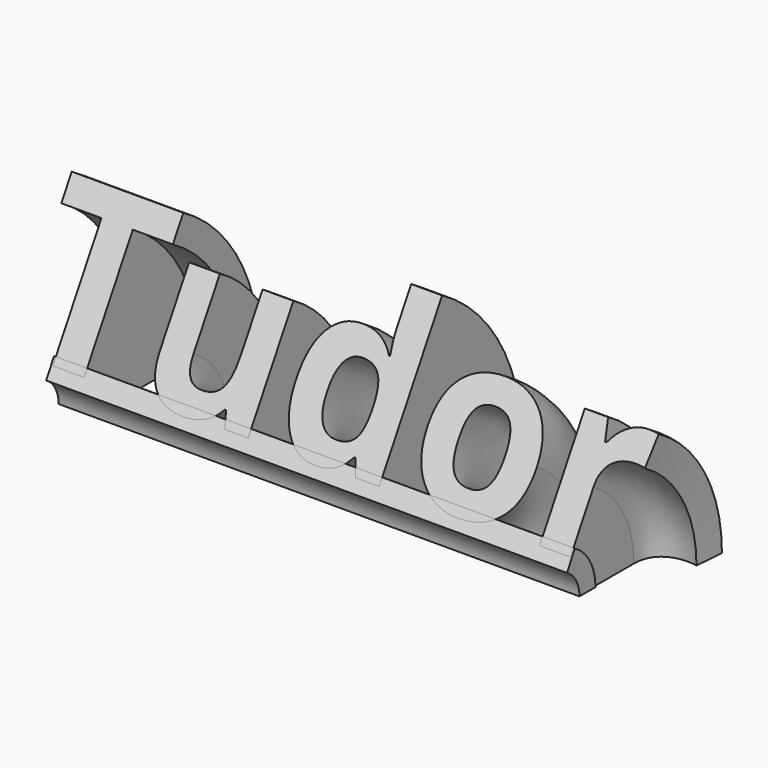
from build123d import *

# Parameters (mm, degrees)
F0_TEXT_SIZE = 44.675252866
F1_W         = 112.4458
F1_H         = 4.3248650618
F3_ANGLE     = 60


# Not quite as in the source:
# - Text() gives the source's letters only with a copy of the font that has no kerning and outlines rounded to 1/6400 em; it was checked with that copy


with BuildPart() as f3:
    # F0 (on Top) + F1 (on Top) → F3 (revolve)
    with BuildSketch(Plane.XY):
        with Locations((-75.3472596407, -8.5821533576)):
            Text('Tudor', F0_TEXT_SIZE, font='Open Sans', font_style=FontStyle.BOLD, text_align=(TextAlign.LEFT, TextAlign.BOTTOM))
    with BuildSketch(Plane.XY):
        with Locations((-9.9333293704, -9.1227616649)):
            Rectangle(F1_W, F1_H)
    revolve(axis=Axis((-0.3378838301, -18.0427953601, 0), (1, 0, 0)), revolution_arc=F3_ANGLE)


solid = f3.part
